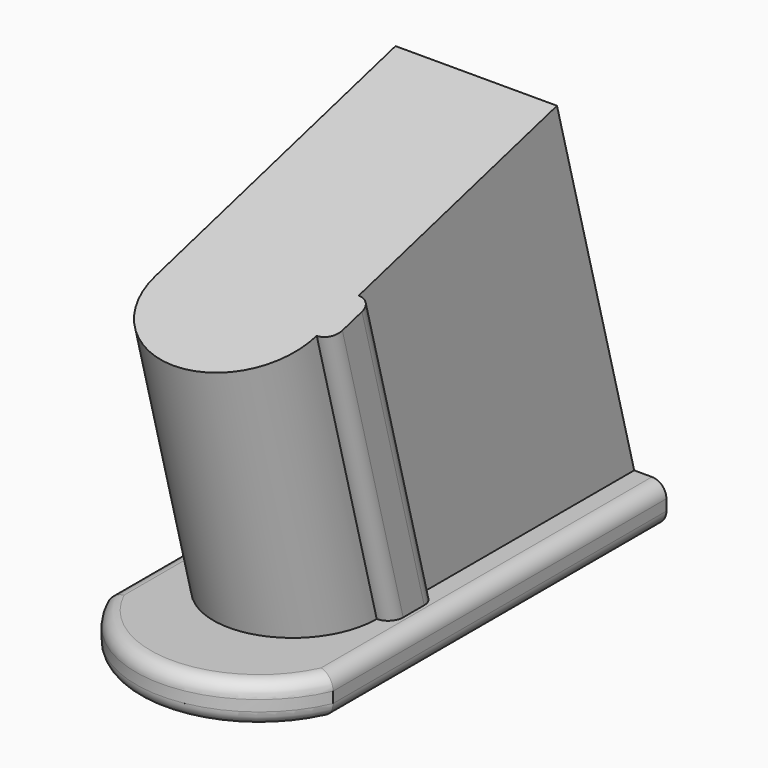
from build123d import *

# Parameters (mm, degrees)
F2_W         = 1
F2_H         = 3.75
F3_DEPTH     = 20
F0_W         = 11.15
F0_H         = 22.225
F0_H_2       = 6.0527027428
F4_DEPTH     = 25
F5_DEPTH     = 2.75
F6_T1_DEPTH  = 33.7778691508
F6_T4_ANGLE  = 166.9020242579
F6_T6_ANGLE  = 166.9020242579
F6_T10_DEPTH = 25
F6_T15_DEPTH = 26.0048094716


# Not quite as in the source:
# - a fillet or chamfer that OpenCascade refuses, or shapes differently, is made with other operations: its cross-section is extruded or revolved along the edge and cut away or added


with BuildPart() as f3:
    # F2 (on line) → F3 (new body, symmetric)
    with BuildSketch(Plane(origin=(0, -0.3533579975, 1.31875), x_dir=(1, 0, 0), z_dir=(0, 0.2588190451, -0.9659258263))):
        with BuildLine():
            ThreePointArc((5.575, 5.0952587337), (0, 10.6702587337), (-5.575, 5.0952587337))
            Line((-5.575, 5.0952587337), (5.575, 5.0952587337))
        make_face()
        Polygon((5.575, 5.0952587337), (-5.575, 5.0952587337), (-5.575, -16.3724427556), (5.575, -16.3724427556), (5.575, 1.3452587337), align=None)
        with Locations((6.075, 3.2202587337)):
            Rectangle(F2_W, F2_H)
    extrude(amount=F3_DEPTH, both=True)

    # F0 (on Top) → F4 (cut)
    with BuildSketch(Plane.XY):
        with BuildLine():
            Line((5.575, -5.275), (-5.575, -5.275))
            ThreePointArc((-5.575, -5.275), (0, -10.85), (5.575, -5.275))
        make_face()
        with BuildLine():
            Line((-5.575, 16.95), (-7.8, 16.95))
            Line((-7.8, 16.95), (-7.8, -11.8278691508))
            ThreePointArc((-7.8, -11.8278691508), (-4.6657321086, -15.5549942921), (0, -16.95))
            ThreePointArc((0, -16.95), (4.6657321086, -15.5549942921), (7.8, -11.8278691508))
            Line((7.8, -11.8278691508), (7.8, 16.95))
            Line((7.8, 16.95), (5.575, 16.95))
            Line((5.575, 16.95), (5.575, -5.275))
            ThreePointArc((5.575, -5.275), (0, -10.85), (-5.575, -5.275))
            Line((-5.575, -5.275), (-5.575, 16.95))
        make_face()
        with Locations((0, 5.8375)):
            Rectangle(F0_W, F0_H)
        with Locations((0, 19.9763513714)):
            Rectangle(F0_W, F0_H_2)
    extrude(amount=-F4_DEPTH, mode=Mode.SUBTRACT)

    # F0 (on Top) → F5 (join)
    with BuildSketch(Plane.XY):
        with BuildLine():
            Line((-5.575, 16.95), (-7.8, 16.95))
            Line((-7.8, 16.95), (-7.8, -11.8278691508))
            ThreePointArc((-7.8, -11.8278691508), (-4.6657321086, -15.5549942921), (0, -16.95))
            ThreePointArc((0, -16.95), (4.6657321086, -15.5549942921), (7.8, -11.8278691508))
            Line((7.8, -11.8278691508), (7.8, 16.95))
            Line((7.8, 16.95), (5.575, 16.95))
            Line((5.575, 16.95), (5.575, -5.275))
            ThreePointArc((5.575, -5.275), (0, -10.85), (-5.575, -5.275))
            Line((-5.575, -5.275), (-5.575, 16.95))
        make_face()
        with BuildLine():
            Line((5.575, -5.275), (-5.575, -5.275))
            ThreePointArc((-5.575, -5.275), (0, -10.85), (5.575, -5.275))
        make_face()
        with Locations((0, 5.8375)):
            Rectangle(F0_W, F0_H)
    extrude(amount=-F5_DEPTH)

    # F6: fillet of radius 1 on 8 edges, made by hand

    # F6_s2 → F6_t1 (cut)
    with BuildSketch(Plane.XZ.offset(-19.45)):
        with BuildLine():
            ThreePointArc((6.8, 0), (7.5071067812, -0.2928932188), (7.8, -1))
            Line((7.8, -1), (7.8, 0))
            Line((7.8, 0), (6.8, 0))
        make_face()
        with BuildLine():
            ThreePointArc((6.8, -2.75), (7.5071067812, -2.4571067812), (7.8, -1.75))
            Line((7.8, -1.75), (7.8, -2.75))
            Line((7.8, -2.75), (6.8, -2.75))
        make_face()
        with BuildLine():
            ThreePointArc((-7.8, -1), (-7.5071067812, -0.2928932188), (-6.8, 0))
            Line((-6.8, 0), (-7.8, 0))
            Line((-7.8, 0), (-7.8, -1))
        make_face()
        with BuildLine():
            ThreePointArc((-7.8, -1.75), (-7.5071067812, -2.4571067812), (-6.8, -2.75))
            Line((-6.8, -2.75), (-7.8, -2.75))
            Line((-7.8, -2.75), (-7.8, -1.75))
        make_face()
    extrude(amount=F6_T1_DEPTH, mode=Mode.SUBTRACT)

    # F6_s3 → F6_t4 (revolve, cut)
    with BuildSketch(Plane(origin=(0.9574563888, -8.3400822912, 0), x_dir=(0, 0, 1), z_dir=(-0.1140526759, 0.9934747038, 0))):
        with BuildLine():
            ThreePointArc((-1, -9.4637451111), (-0.2928932188, -9.1708518923), (0, -8.4637451111))
            Line((0, -8.4637451111), (0, -9.4637451111))
            Line((0, -9.4637451111), (-1, -9.4637451111))
        make_face()
    revolve(axis=Axis((0, -8.45, 0), (0, 0, 1)), revolution_arc=F6_T4_ANGLE, mode=Mode.SUBTRACT)

    # F6_s5 → F6_t6 (revolve, cut)
    with BuildSketch(Plane(origin=(0.9574563888, -8.3400822912, 0), x_dir=(0, 0, 1), z_dir=(-0.1140526759, 0.9934747038, 0))):
        with BuildLine():
            ThreePointArc((-1.75, -9.4637451111), (-2.4571067812, -9.1708518923), (-2.75, -8.4637451111))
            Line((-2.75, -8.4637451111), (-2.75, -9.4637451111))
            Line((-2.75, -9.4637451111), (-1.75, -9.4637451111))
        make_face()
    revolve(axis=Axis((0, -8.45, -2.75), (0, 0, 1)), revolution_arc=F6_T6_ANGLE, mode=Mode.SUBTRACT)


with BuildPart() as f6_tool8:
    # F6_s9 → F6_t10 (new body)
    with BuildSketch(Plane(origin=(0, 0.2936896152, -1.0960645657), x_dir=(1, 0, 0), z_dir=(0, -0.2588190451, 0.9659258263))):
        with BuildLine():
            ThreePointArc((5.575, -5.0952587337), (6.2821067812, -4.8023655149), (6.575, -4.0952587337))
            Line((6.575, -4.0952587337), (6.575, -5.0952587337))
            Line((6.575, -5.0952587337), (5.575, -5.0952587337))
        make_face()
    extrude(amount=F6_T10_DEPTH)

    split(bisect_by=Plane.XY, keep=Keep.TOP)


with BuildPart() as f3_1:
    add(f3.part)

    # F6_t7: cut F6_tool8
    add(f6_tool8.part, mode=Mode.SUBTRACT)


with BuildPart() as f6_tool13:
    # F6_s14 → F6_t15 (new body)
    with BuildSketch(Plane(origin=(0, 0.5537534432, -2.0666359849), x_dir=(1, 0, 0), z_dir=(0, -0.2588190451, 0.9659258263))):
        with BuildLine():
            ThreePointArc((6.575, -2.3452587337), (6.2821067812, -1.6381519525), (5.575, -1.3452587337))
            Line((5.575, -1.3452587337), (6.575, -1.3452587337))
            Line((6.575, -1.3452587337), (6.575, -2.3452587337))
        make_face()
    extrude(amount=F6_T15_DEPTH)

    split(bisect_by=Plane.XY, keep=Keep.TOP)


with BuildPart() as f3_2:
    add(f3_1.part)

    # F6_t12: cut F6_tool13
    add(f6_tool13.part, mode=Mode.SUBTRACT)


solid = f3_2.part
